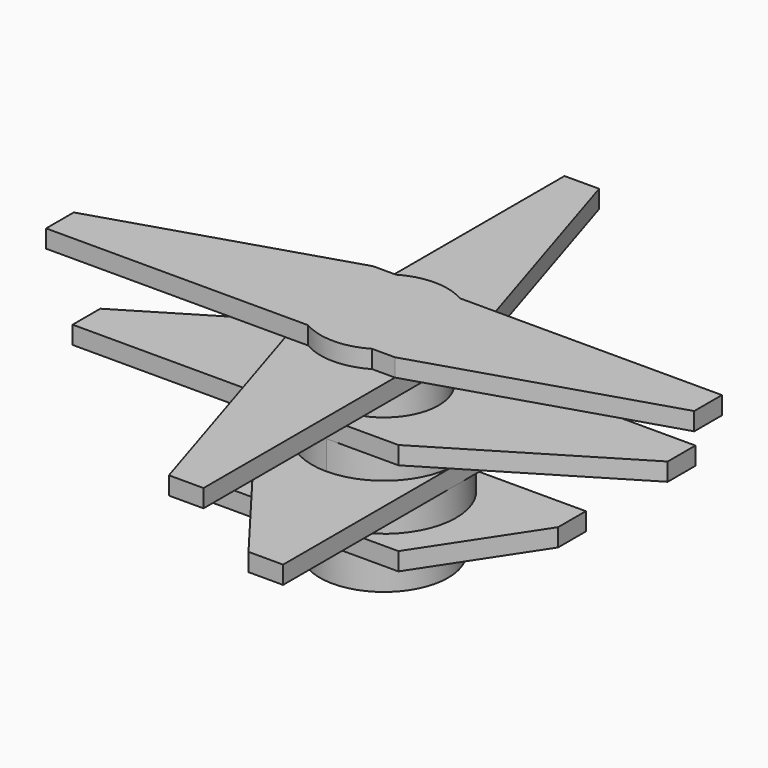
from build123d import *

# Parameters (mm, degrees)
F1_DEPTH  = 6.2
F3_DEPTH  = 6.2
F5_DEPTH  = 10
F6_W      = 50
F6_H      = 50
F6_R      = 19
F7_DEPTH  = 6.2
F9_DEPTH  = 10
F11_DEPTH = 6.2
F13_DEPTH = 10
F15_DEPTH = 6.2
F16_R     = 22.25
F17_DEPTH = 13
F19_D     = 35
F19_DEPTH = 35
F19_TIP   = 10.515060833


with BuildPart() as f1:
    # F0 (on Top) → F1 (new body)
    with BuildSketch(Plane.XY):
        with BuildLine():
            Line((102, 19), (11.0905365064, 19))
            ThreePointArc((11.0905365064, 19), (0, 22), (-11.0905365064, 19))
            Line((-11.0905365064, 19), (-19, 19))
            Line((-19, 19), (-102, -7))
            Line((-102, -7), (-102, -19))
            Line((-102, -19), (-11.0905365064, -19))
            ThreePointArc((-11.0905365064, -19), (0, -22), (11.0905365064, -19))
            Line((11.0905365064, -19), (19, -19))
            Line((19, -19), (102, 7))
            Line((102, 7), (102, 19))
        make_face()
    extrude(amount=F1_DEPTH)

    # F2 (on face) → F3 (join)
    with BuildSketch(Plane(origin=(0, 0, 0), x_dir=(1, 0, 0), z_dir=(0, 0, -1))):
        with BuildLine():
            Line((-19, 19), (-19, 0))
            Line((-19, 0), (-19, -19))
            Line((-19, -19), (-11.0905365064, -19))
            ThreePointArc((-11.0905365064, -19), (0, -22), (11.0905365064, -19))
            Line((11.0905365064, -19), (19, -19))
            Line((19, -19), (19, 0))
            Line((19, 0), (19, 19))
            Line((19, 19), (11.0905365064, 19))
            ThreePointArc((11.0905365064, 19), (0, 22), (-11.0905365064, 19))
            Line((-11.0905365064, 19), (-19, 19))
        make_face()
        with BuildLine():
            Line((-11.0905365064, -19), (-19, -19))
            Line((-19, -19), (-19, -102))
            Line((-19, -102), (-7, -102))
            Line((-7, -102), (19, -19))
            Line((19, -19), (11.0905365064, -19))
            ThreePointArc((11.0905365064, -19), (0, -22), (-11.0905365064, -19))
        make_face()
        with BuildLine():
            Line((7, 102), (-19, 19))
            Line((-19, 19), (-11.0905365064, 19))
            ThreePointArc((-11.0905365064, 19), (0, 22), (11.0905365064, 19))
            Line((11.0905365064, 19), (19, 19))
            Line((19, 19), (19, 102))
            Line((19, 102), (7, 102))
        make_face()
    extrude(amount=F3_DEPTH)

    # F4 (on face) → F5 (join)
    with BuildSketch(Plane(origin=(0, 0, -6.2), x_dir=(1, 0, 0), z_dir=(0, 0, -1))):
        with BuildLine():
            ThreePointArc((-19, 0), (0, -19), (19, 0))
            ThreePointArc((19, 0), (0, 19), (-19, 0))
        make_face()
    extrude(amount=F5_DEPTH)

    # F6 (on face) → F7 (join)
    with BuildSketch(Plane(origin=(0, 0, -16.2), x_dir=(1, 0, 0), z_dir=(0, 0, -1))):
        Rectangle(F6_W, F6_H)
        Circle(F6_R, mode=Mode.SUBTRACT)
        Polygon((25, 25), (25, -25), (88, -25), (88, -13), align=None)
        Polygon((-88, 13), (-25, -25), (-25, 25), (-88, 25), align=None)
        Circle(F6_R)
    extrude(amount=F7_DEPTH)

    # F8 (on face) → F9 (join)
    with BuildSketch(Plane(origin=(0, 0, -22.4), x_dir=(1, 0, 0), z_dir=(0, 0, -1))):
        with BuildLine():
            ThreePointArc((-5.83e-08, -25), (17.677669509, -17.6776695503), (25, 0))
            ThreePointArc((25, 0), (17.6776695297, 17.6776695297), (0, 25))
            ThreePointArc((0, 25), (-25, 2.92e-08), (-5.83e-08, -25))
        make_face()
    extrude(amount=F9_DEPTH)

    # F10 (on face) → F11 (join)
    with BuildSketch(Plane(origin=(0, 0, -32.4), x_dir=(1, 0, 0), z_dir=(0, 0, -1))):
        Polygon((13, 75), (-25, 25), (4.22e-08, 25), (25, 25), (25, 75), align=None)
        with BuildLine():
            ThreePointArc((4.22e-08, 25), (17.6776695446, 17.6776695147), (25, 0))
            Line((25, 0), (25, 25))
            Line((25, 25), (4.22e-08, 25))
        make_face()
        with BuildLine():
            ThreePointArc((-25, 0), (-17.6776695332, -17.6776695262), (-9.9e-09, -25))
            ThreePointArc((-9.9e-09, -25), (17.6776695262, -17.6776695332), (25, 0))
            ThreePointArc((25, 0), (17.6776695446, 17.6776695147), (4.22e-08, 25))
            ThreePointArc((4.22e-08, 25), (-17.6776695147, 17.6776695446), (-25, 0))
        make_face()
        with BuildLine():
            ThreePointArc((25, 0), (17.6776695262, -17.6776695332), (-9.9e-09, -25))
            Line((-9.9e-09, -25), (25, -25))
            Line((25, -25), (25, 0))
        make_face()
        Polygon((-9.9e-09, -25), (-25, -25), (-25, -75), (-13, -75), (25, -25), align=None)
        with BuildLine():
            Line((-25, 0), (-25, -25))
            Line((-25, -25), (-9.9e-09, -25))
            ThreePointArc((-9.9e-09, -25), (-17.6776695332, -17.6776695262), (-25, 0))
        make_face()
        with BuildLine():
            Line((-25, 25), (-25, 0))
            ThreePointArc((-25, 0), (-17.6776695147, 17.6776695446), (4.22e-08, 25))
            Line((4.22e-08, 25), (-25, 25))
        make_face()
    extrude(amount=F11_DEPTH)

    # F12 (on face) → F13 (join)
    with BuildSketch(Plane(origin=(0, 0, -38.6), x_dir=(1, 0, 0), z_dir=(0, 0, -1))):
        with BuildLine():
            ThreePointArc((-25, 2.61e-08), (-1.3e-08, -25), (25, 0))
            ThreePointArc((25, 0), (1.3e-08, 25), (-25, 2.61e-08))
        make_face()
    extrude(amount=F13_DEPTH)

    # F14 (on face) → F15 (join)
    with BuildSketch(Plane(origin=(0, 0, -48.6), x_dir=(1, 0, 0), z_dir=(0, 0, -1))):
        with BuildLine():
            ThreePointArc((-25, 0), (-17.6776695204, -17.6776695389), (2.61e-08, -25))
            ThreePointArc((2.61e-08, -25), (17.6776695389, -17.6776695204), (25, 0))
            ThreePointArc((25, 0), (17.6776695389, 17.6776695204), (2.61e-08, 25))
            ThreePointArc((2.61e-08, 25), (-17.6776695204, 17.6776695389), (-25, 0))
        make_face()
        with BuildLine():
            ThreePointArc((2.61e-08, 25), (17.6776695389, 17.6776695204), (25, 0))
            Line((25, 0), (25, 25))
            Line((25, 25), (2.61e-08, 25))
        make_face()
        with BuildLine():
            Line((2.61e-08, -25), (25, -25))
            Line((25, -25), (25, 0))
            ThreePointArc((25, 0), (17.6776695389, -17.6776695204), (2.61e-08, -25))
        make_face()
        with BuildLine():
            Line((-25, -25), (2.61e-08, -25))
            ThreePointArc((2.61e-08, -25), (-17.6776695204, -17.6776695389), (-25, 0))
            Line((-25, 0), (-25, -25))
        make_face()
        with BuildLine():
            Line((-25, 25), (-25, 0))
            ThreePointArc((-25, 0), (-17.6776695204, 17.6776695389), (2.61e-08, 25))
            Line((2.61e-08, 25), (-25, 25))
        make_face()
        Polygon((-50, 13), (-25, -25), (-25, 0), (-25, 25), (-50, 25), align=None)
        Polygon((25, 0), (25, -25), (50, -25), (50, -13), (25, 25), align=None)
    extrude(amount=F15_DEPTH)

    # F16 (on face) → F17 (join)
    with BuildSketch(Plane(origin=(0, 0, -54.8), x_dir=(1, 0, 0), z_dir=(0, 0, -1))):
        Circle(F16_R)
    extrude(amount=F17_DEPTH)

    # F19
    with Locations(Plane(origin=(0, 0, -67.8), x_dir=(1, 0, 0), z_dir=(0, 0, -1))):
        with Locations((0, 0)):
            Hole(F19_D / 2, depth=F19_DEPTH)
            with Locations((0, 0, -(F19_DEPTH + F19_TIP / 2))):  # 118° drill point
                Cone(0, F19_D / 2, F19_TIP, mode=Mode.SUBTRACT)


solid = f1.part
